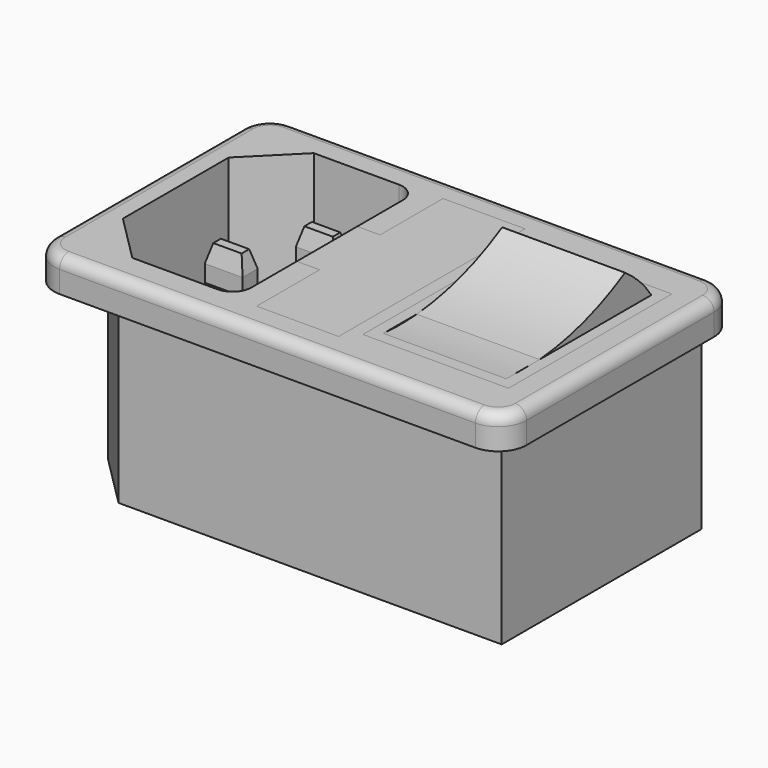
from build123d import *

# Parameters (mm, degrees)
F0_W        = 15.4
F0_H        = 21.6
F1_DEPTH    = 3.5
F0_W_2      = 4
F0_H_2      = 2
F0_W_3      = 13
F0_H_3      = 19.2
F0_W_4      = 2.418700546
F0_H_4      = 8
F2_DEPTH    = 19
F3_DEPTH    = 15
F4_C1_SIZE2 = 0.5
F4_C1_SIZE  = 1.8660254038
F4_C2_SIZE2 = 0.5
F4_C2_SIZE  = 1.8660254038
F4_C3_SIZE2 = 1.8660254038
F4_C3_SIZE  = 0.5
F4_C4_SIZE2 = 1.8660254038
F4_C4_SIZE  = 0.5
F5_SIZE2    = 1.8660254038
F5_SIZE     = 0.5
F6_SIZE2    = 1.8660254038
F6_SIZE     = 0.5
F7_DEPTH    = 3.5
F8_DEPTH    = 22
F10_DEPTH   = 25
F11_R       = 1.2


with BuildPart() as f1:
    # F0 (on Top) → F1 (new body)
    with BuildSketch(Plane.XY):
        with BuildLine():
            Line((21.4106866419, 15.232257545), (-22.5893133581, 15.232257545))
            ThreePointArc((-22.5893133581, 15.232257545), (-24.7106337016, 14.3535778886), (-25.5893133581, 12.232257545))
            Line((-25.5893133581, 12.232257545), (-25.5893133581, -12.567742455))
            ThreePointArc((-25.5893133581, -12.567742455), (-24.7106337016, -14.6890627986), (-22.5893133581, -15.567742455))
            Line((-22.5893133581, -15.567742455), (21.4106866419, -15.567742455))
            ThreePointArc((21.4106866419, -15.567742455), (23.5320069855, -14.6890627986), (24.4106866419, -12.567742455))
            Line((24.4106866419, -12.567742455), (24.4106866419, 12.232257545))
            ThreePointArc((24.4106866419, 12.232257545), (23.5320069855, 14.3535778886), (21.4106866419, 15.232257545))
        make_face()
        Polygon((-18.2525572471, 13.2), (-8.7555009723, 13.2), (22.2888856925, 13.2), (22.2888856925, -13.2), (-8.7555009723, -13.2), (-18.2525572471, -13.2), (-23.9555009723, -7.4970562748), (-23.9555009723, 7.4970562748), align=None, mode=Mode.SUBTRACT)
        Polygon((22.2888856925, 13.2), (-8.7555009723, 13.2), (-18.2525572471, 13.2), (-23.9555009723, 7.4970562748), (-23.9555009723, -7.4970562748), (-18.2525572471, -13.2), (-8.7555009723, -13.2), (22.2888856925, -13.2), align=None)
        with BuildLine():
            Line((-4.3368004262, 4), (-4.3368004262, 12.3322419822))
            Line((-4.3368004262, 12.3322419822), (4.3368004262, 12.3322419822))
            Line((4.3368004262, 12.3322419822), (4.3368004262, -12.3322419822))
            Line((4.3368004262, -12.3322419822), (-4.3368004262, -12.3322419822))
            Line((-4.3368004262, -12.3322419822), (-4.3368004262, -4))
            Line((-4.3368004262, -4), (-6.7555009723, -4))
            Line((-6.7555009723, -4), (-6.7555009723, -10))
            ThreePointArc((-6.7555009723, -10), (-7.3412874099, -11.4142135624), (-8.7555009723, -12))
            Line((-8.7555009723, -12), (-17.7555009723, -12))
            Line((-17.7555009723, -12), (-22.7555009723, -7))
            Line((-22.7555009723, -7), (-22.7555009723, 7))
            Line((-22.7555009723, 7), (-17.7555009723, 12))
            Line((-17.7555009723, 12), (-8.7555009723, 12))
            ThreePointArc((-8.7555009723, 12), (-7.3412874099, 11.4142135624), (-6.7555009723, 10))
            Line((-6.7555009723, 10), (-6.7555009723, 4))
            Line((-6.7555009723, 4), (-4.3368004262, 4))
        make_face(mode=Mode.SUBTRACT)
        with Locations((13.3888856925, 0)):
            Rectangle(F0_W, F0_H, mode=Mode.SUBTRACT)
    extrude(amount=F1_DEPTH)

    # F0 (on Top) → F2 (join)
    with BuildSketch(Plane.XY):
        Polygon((22.2888856925, 13.2), (-8.7555009723, 13.2), (-18.2525572471, 13.2), (-23.9555009723, 7.4970562748), (-23.9555009723, -7.4970562748), (-18.2525572471, -13.2), (-8.7555009723, -13.2), (22.2888856925, -13.2), align=None)
        with BuildLine():
            Line((-4.3368004262, 4), (-4.3368004262, 12.3322419822))
            Line((-4.3368004262, 12.3322419822), (4.3368004262, 12.3322419822))
            Line((4.3368004262, 12.3322419822), (4.3368004262, -12.3322419822))
            Line((4.3368004262, -12.3322419822), (-4.3368004262, -12.3322419822))
            Line((-4.3368004262, -12.3322419822), (-4.3368004262, -4))
            Line((-4.3368004262, -4), (-6.7555009723, -4))
            Line((-6.7555009723, -4), (-6.7555009723, -10))
            ThreePointArc((-6.7555009723, -10), (-7.3412874099, -11.4142135624), (-8.7555009723, -12))
            Line((-8.7555009723, -12), (-17.7555009723, -12))
            Line((-17.7555009723, -12), (-22.7555009723, -7))
            Line((-22.7555009723, -7), (-22.7555009723, 7))
            Line((-22.7555009723, 7), (-17.7555009723, 12))
            Line((-17.7555009723, 12), (-8.7555009723, 12))
            ThreePointArc((-8.7555009723, 12), (-7.3412874099, 11.4142135624), (-6.7555009723, 10))
            Line((-6.7555009723, 10), (-6.7555009723, 4))
            Line((-6.7555009723, 4), (-4.3368004262, 4))
        make_face(mode=Mode.SUBTRACT)
        with Locations((13.3888856925, 0)):
            Rectangle(F0_W, F0_H, mode=Mode.SUBTRACT)
        with BuildLine():
            Line((-6.7555009723, -4), (-6.7555009723, 4))
            Line((-6.7555009723, 4), (-6.7555009723, 10))
            ThreePointArc((-6.7555009723, 10), (-7.3412874099, 11.4142135624), (-8.7555009723, 12))
            Line((-8.7555009723, 12), (-17.7555009723, 12))
            Line((-17.7555009723, 12), (-22.7555009723, 7))
            Line((-22.7555009723, 7), (-22.7555009723, -7))
            Line((-22.7555009723, -7), (-17.7555009723, -12))
            Line((-17.7555009723, -12), (-8.7555009723, -12))
            ThreePointArc((-8.7555009723, -12), (-7.3412874099, -11.4142135624), (-6.7555009723, -10))
            Line((-6.7555009723, -10), (-6.7555009723, -4))
        make_face()
        with Locations((-12.8875139207, -6.9733052514)):
            Rectangle(F0_W_2, F0_H_2, mode=Mode.SUBTRACT)
        with Locations((-16.8875139207, 0)):
            Rectangle(F0_W_2, F0_H_2, mode=Mode.SUBTRACT)
        with Locations((-12.8875139207, 7.0500936662)):
            Rectangle(F0_W_2, F0_H_2, mode=Mode.SUBTRACT)
        with Locations((13.3888856925, 0)):
            Rectangle(F0_W, F0_H)
        with Locations((13.3888856925, 0)):
            Rectangle(F0_W_3, F0_H_3, mode=Mode.SUBTRACT)
        with Locations((13.3888856925, 0)):
            Rectangle(F0_W_3, F0_H_3)
        Polygon((4.3368004262, 12.3322419822), (-4.3368004262, 12.3322419822), (-4.3368004262, 4), (-4.3368004262, -4), (-4.3368004262, -12.3322419822), (4.3368004262, -12.3322419822), align=None)
        with Locations((-5.5461506993, 0)):
            Rectangle(F0_W_4, F0_H_4)
        with Locations((-12.8875139207, -6.9733052514)):
            Rectangle(F0_W_2, F0_H_2)
        with Locations((-16.8875139207, 0)):
            Rectangle(F0_W_2, F0_H_2)
        with Locations((-12.8875139207, 7.0500936662)):
            Rectangle(F0_W_2, F0_H_2)
    extrude(amount=-F2_DEPTH)

    # F0 (on Top) → F3 (cut)
    with BuildSketch(Plane.XY):
        with BuildLine():
            Line((-6.7555009723, -4), (-6.7555009723, 4))
            Line((-6.7555009723, 4), (-6.7555009723, 10))
            ThreePointArc((-6.7555009723, 10), (-7.3412874099, 11.4142135624), (-8.7555009723, 12))
            Line((-8.7555009723, 12), (-17.7555009723, 12))
            Line((-17.7555009723, 12), (-22.7555009723, 7))
            Line((-22.7555009723, 7), (-22.7555009723, -7))
            Line((-22.7555009723, -7), (-17.7555009723, -12))
            Line((-17.7555009723, -12), (-8.7555009723, -12))
            ThreePointArc((-8.7555009723, -12), (-7.3412874099, -11.4142135624), (-6.7555009723, -10))
            Line((-6.7555009723, -10), (-6.7555009723, -4))
        make_face()
        with Locations((-12.8875139207, -6.9733052514)):
            Rectangle(F0_W_2, F0_H_2, mode=Mode.SUBTRACT)
        with Locations((-16.8875139207, 0)):
            Rectangle(F0_W_2, F0_H_2, mode=Mode.SUBTRACT)
        with Locations((-12.8875139207, 7.0500936662)):
            Rectangle(F0_W_2, F0_H_2, mode=Mode.SUBTRACT)
        with Locations((13.3888856925, 0)):
            Rectangle(F0_W_3, F0_H_3)
    extrude(amount=-F3_DEPTH, mode=Mode.SUBTRACT)

    # F4: chamfer of 0.5 x 1.8660254038 on 4 edges, made by hand

    # F4_c1
    f4_c1_edges = [f1.edges().sort_by_distance(p)[0] for p in [
        (-10.8875139207, 7.0500936662, 0),
    ]]
    f4_c1_side = f1.faces().sort_by_distance((-10.8875139207, 7.0500936662, -0.01))[0]
    chamfer(f4_c1_edges, length=F4_C1_SIZE, length2=F4_C1_SIZE2, reference=f4_c1_side)

    # F4_c2
    f4_c2_edges = [f1.edges().sort_by_distance(p)[0] for p in [
        (-13.1375139207, 6.0500936662, 0),
    ]]
    f4_c2_side = f1.faces().sort_by_distance((-13.1375139207, 6.0500936662, -0.01))[0]
    chamfer(f4_c2_edges, length=F4_C2_SIZE, length2=F4_C2_SIZE2, reference=f4_c2_side)

    # F4_c3
    f4_c3_edges = [f1.edges().sort_by_distance(p)[0] for p in [
        (-14.8875139207, 7.3000936662, 0),
    ]]
    f4_c3_side = f1.faces().sort_by_distance((-14.8775139207, 7.3000936662, 0))[0]
    chamfer(f4_c3_edges, length=F4_C3_SIZE, length2=F4_C3_SIZE2, reference=f4_c3_side)

    # F4_c4
    f4_c4_edges = [f1.edges().sort_by_distance(p)[0] for p in [
        (-12.8875139207, 8.0500936662, 0),
    ]]
    f4_c4_side = f1.faces().sort_by_distance((-12.8875139207, 8.0400936662, 0))[0]
    chamfer(f4_c4_edges, length=F4_C4_SIZE, length2=F4_C4_SIZE2, reference=f4_c4_side)

    # F5
    f5_edges = [f1.edges().sort_by_distance(p)[0] for p in [
        (-16.887514, 1, 0),
        (-14.887514, 0, 0),
        (-16.887514, -1, 0),
        (-18.887514, 0, 0),
    ]]
    f5_side = f1.faces().sort_by_distance((-16.887514, 0, 0))[0]
    chamfer(f5_edges, length=F5_SIZE, length2=F5_SIZE2, reference=f5_side)

    # F6
    f6_edges = [f1.edges().sort_by_distance(p)[0] for p in [
        (-14.887514, -6.973305, 0),
        (-12.887514, -5.973305, 0),
        (-10.887514, -6.973305, 0),
        (-12.887514, -7.973305, 0),
    ]]
    f6_side = f1.faces().sort_by_distance((-12.887514, -6.973305, 0))[0]
    chamfer(f6_edges, length=F6_SIZE, length2=F6_SIZE2, reference=f6_side)


with BuildPart() as f7:
    # F7 (new, through all): a face of the model
    f7_faces = [f1.part.faces().sort_by_distance(p)[0] for p in [
        (-0.4600310991, 0, 0),
    ]]
    extrude(f7_faces, amount=F7_DEPTH)


with BuildPart() as f7b:
    # F7#2 (new, through all): a face of the model
    f7_2_faces = [f1.part.faces().sort_by_distance(p)[0] for p in [
        (13.3888856925, -10.5347227865, 0),
    ]]
    extrude(f7_2_faces, amount=F7_DEPTH)


with BuildPart() as f8:
    # F8 (new): a face of the model
    f8_faces = [f1.part.faces().sort_by_distance(p)[0] for p in [
        (13.3888856925, 0, -15),
    ]]
    extrude(f8_faces, amount=F8_DEPTH)

    # F9 (on face) → F10 (cut)
    with BuildSketch(Plane.YZ.offset(19.8888856925)):
        with BuildLine():
            ThreePointArc((-9.6, 3.5), (-7.3938840069, 3.410434439), (-5.1877680138, 3.5))
            Line((-5.1877680138, 3.5), (-9.6, 3.5))
        make_face()
        with BuildLine():
            Line((-9.6, 3.5), (-5.1877680138, 3.5))
            ThreePointArc((-5.1877680138, 3.5), (0.6561669902, 4.6282852574), (6.1150655176, 7))
            Line((6.1150655176, 7), (-9.6, 7))
            Line((-9.6, 7), (-9.6, 3.5))
        make_face()
        with BuildLine():
            ThreePointArc((6.1150655176, 7), (8.0179372576, 5.4097140483), (9.6, 3.5))
            Line((9.6, 3.5), (9.6, 7))
            Line((9.6, 7), (6.1150655176, 7))
        make_face()
    extrude(amount=-F10_DEPTH, mode=Mode.SUBTRACT)


with BuildPart() as f1_1:
    add(f1.part)

    # F11
    f11_edges = [f1_1.edges().sort_by_distance(p)[0] for p in [
        (-25.589313, -0.167742, 3.5),
        (24.410687, -0.167742, 3.5),
        (23.532007, 14.353578, 3.5),
        (-0.589313, 15.232258, 3.5),
        (-24.710634, 14.353578, 3.5),
        (-24.710634, -14.689063, 3.5),
        (-0.589313, -15.567742, 3.5),
        (23.532007, -14.689063, 3.5),
    ]]
    fillet(f11_edges, radius=F11_R)


solid = Compound([f7.part, f7b.part, f8.part, f1_1.part])
